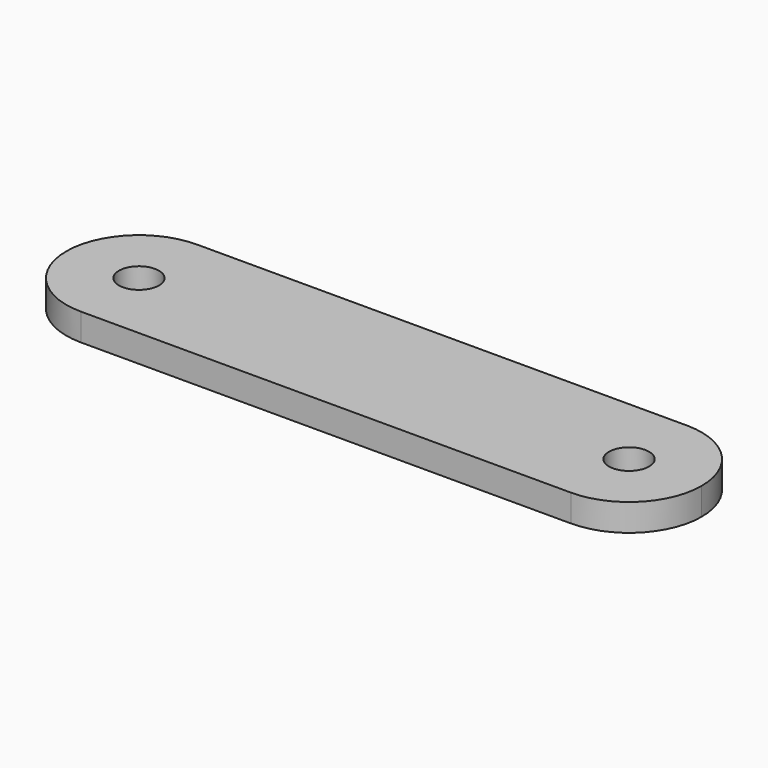
from build123d import *

# Parameters (mm, degrees)
F0_W     = 111.125
F0_H     = 25.4
F1_DEPTH = 4.7498
F2_R     = 12.69999
F3_R     = 3.5
F3_R_2   = 3.5052
F4_DEPTH = 25.4


# Not quite as in the source:
# - a fillet or chamfer is up to 0.001 mm smaller than in the source, because OpenCascade refuses the exact size


with BuildPart() as f1:
    # F0 (on Top) → F1 (new body)
    with BuildSketch(Plane.XY):
        Rectangle(F0_W, F0_H)
    extrude(amount=F1_DEPTH)

    # F2 (radius 12.7 in the source; OpenCascade refuses exactly that, so slightly less here)
    f2_edges = [f1.edges().sort_by_distance(p)[0] for p in [
        (-55.5625, -12.7, 2.3749),
        (-55.5625, 12.7, 2.3749),
        (55.5625, -12.7, 2.3749),
        (55.5625, 12.7, 2.3749),
    ]]
    fillet(f2_edges, radius=F2_R)

    # F3 (on face) → F4 (cut)
    with BuildSketch(Plane.XY.offset(4.7498)):
        with Locations((-42.8625, 0)):
            Circle(F3_R)
        with Locations((42.8625, 0)):
            Circle(F3_R_2)
    extrude(amount=-F4_DEPTH, mode=Mode.SUBTRACT)


solid = f1.part
